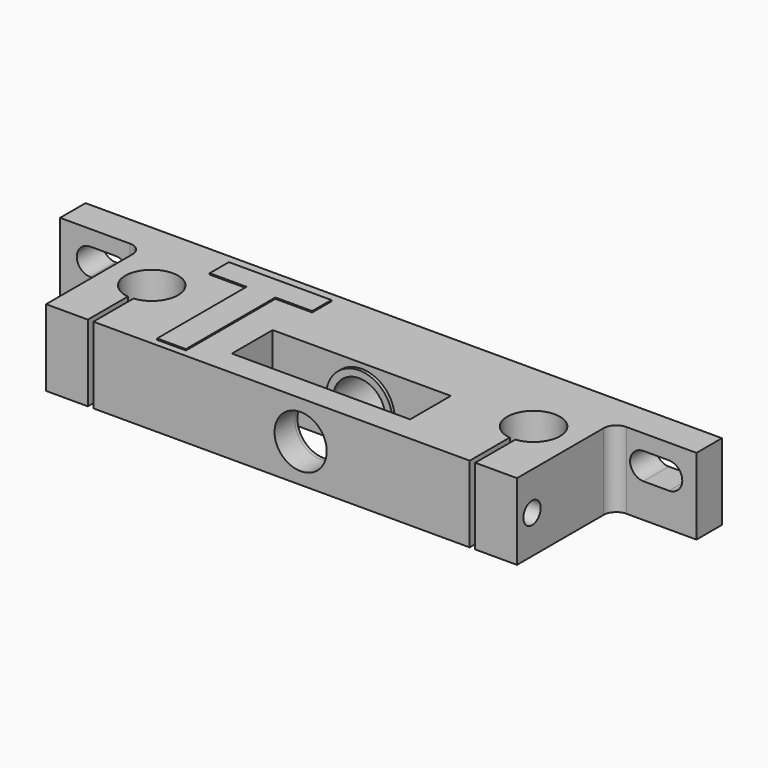
from build123d import *
from build123d import SkipClean  # not in build123d's __all__

# Parameters (mm, degrees)
F1_DEPTH      = 12
F3_DEPTH      = 12.001
F5_DEPTH      = 24.001
F6_R          = 4.1
F7_DEPTH      = 20
F8_W          = 14
F8_H          = 8
F9_DEPTH      = 12.001
F10_R         = 5.1951476321
F10_R_2       = 4.1
F11_DEPTH     = 0.5
F12_R         = 5.2529872518
F12_R_2       = 4.1
F13_DEPTH     = 0.5
F14_TEXT_SIZE = 29.872882718
F15_DEPTH     = 0.2
F16_R         = 1.4
F17_DEPTH     = 18
F16_R_2       = 1.7
F18_DEPTH     = 6.5630027184
F19_R         = 2
F20_R         = 1.4
F21_DEPTH     = 18
F20_R_2       = 1.7
F22_DEPTH     = 6.5630027184
F23_R         = 2


# Not quite as in the source:
# - after a boolean that leaves OpenCascade's solid faulty, fix() repairs it
# - Text() gives the source's letters only with a copy of the font that has no kerning and outlines rounded to 1/6400 em; it was checked with that copy


with BuildPart() as f1:
    # F0 (on Top) → F1 (new body)
    with BuildSketch(Plane.XY):
        Polygon((53.6500561982, 12.3083528318), (-46.3499438018, 12.3083528318), (-46.3499438018, 7.3083528318), (-33.3499438018, 7.3083528318), (-33.3499438018, -11.6916471682), (40.6500561982, -11.6916471682), (40.6500561982, 7.3083528318), (53.6500561982, 7.3083528318), align=None)
    extrude(amount=F1_DEPTH)

    # F2 (on face) → F3 (cut, through all)
    with BuildSketch(Plane.XY.offset(12)):
        with BuildLine():
            ThreePointArc((-25.9119465202, -3.818468994), (-23.2644787867, -2.4669679859), (-22.1999438018, 0.3083528318))
            ThreePointArc((-22.1999438018, 0.3083528318), (-29.1252646194, 3.3938178468), (-26.7879410833, -3.818468994))
            Line((-26.7879410833, -3.818468994), (-26.7879410833, -3.0108469723))
            Line((-26.7879410833, -3.0108469723), (-25.9119465202, -3.0108469723))
            Line((-25.9119465202, -3.0108469723), (-25.9119465202, -3.818468994))
        make_face()
        with BuildLine():
            Line((-26.7879410833, -3.0108469723), (-26.7879410833, -3.818468994))
            ThreePointArc((-26.7879410833, -3.818468994), (-26.3499438018, -3.8416471682), (-25.9119465202, -3.818468994))
            Line((-25.9119465202, -3.818468994), (-25.9119465202, -3.0108469723))
            Line((-25.9119465202, -3.0108469723), (-26.7879410833, -3.0108469723))
        make_face()
        with BuildLine():
            ThreePointArc((-25.9119465202, -3.818468994), (-26.3499438018, -3.8416471682), (-26.7879410833, -3.818468994))
            Line((-26.7879410833, -3.818468994), (-26.7879410833, -12.2696550748))
            Line((-26.7879410833, -12.2696550748), (-25.9119465202, -12.2696550748))
            Line((-25.9119465202, -12.2696550748), (-25.9119465202, -3.818468994))
        make_face()
        with BuildLine():
            ThreePointArc((34.0880534798, -3.818468994), (36.7355212133, -2.4669679859), (37.8000561982, 0.3083528318))
            ThreePointArc((37.8000561982, 0.3083528318), (30.8747353806, 3.3938178468), (33.2120589167, -3.818468994))
            Line((33.2120589167, -3.818468994), (33.2120589167, -3.0108469723))
            Line((33.2120589167, -3.0108469723), (34.0880534798, -3.0108469723))
            Line((34.0880534798, -3.0108469723), (34.0880534798, -3.818468994))
        make_face()
        with BuildLine():
            Line((33.2120589167, -3.0108469723), (33.2120589167, -3.818468994))
            ThreePointArc((33.2120589167, -3.818468994), (33.6500561982, -3.8416471682), (34.0880534798, -3.818468994))
            Line((34.0880534798, -3.818468994), (34.0880534798, -3.0108469723))
            Line((34.0880534798, -3.0108469723), (33.2120589167, -3.0108469723))
        make_face()
        with BuildLine():
            ThreePointArc((34.0880534798, -3.818468994), (33.6500561982, -3.8416471682), (33.2120589167, -3.818468994))
            Line((33.2120589167, -3.818468994), (33.2120589167, -12.2696550748))
            Line((33.2120589167, -12.2696550748), (34.0880534798, -12.2696550748))
            Line((34.0880534798, -12.2696550748), (34.0880534798, -3.818468994))
        make_face()
    extrude(amount=-F3_DEPTH, mode=Mode.SUBTRACT)

    # F4 (on face) → F5 (cut, through all)
    with BuildSketch(Plane(origin=(0, 12.3083528318, 0), x_dir=(-1, 0, 0), z_dir=(0, 1, 0))):
        with BuildLine():
            Line((-45.3214800954, 9.5596171677), (-49.3214800954, 9.5596171677))
            ThreePointArc((-49.3214800954, 9.5596171677), (-51.4214800954, 7.4596171677), (-49.3214800954, 5.3596171677))
            Line((-49.3214800954, 5.3596171677), (-45.3214800954, 5.3596171677))
            ThreePointArc((-45.3214800954, 5.3596171677), (-43.2214800954, 7.4596171677), (-45.3214800954, 9.5596171677))
        make_face()
        with BuildLine():
            ThreePointArc((37.6219116151, 9.5596171677), (35.5219116151, 7.4596171677), (37.6219116151, 5.3596171677))
            Line((37.6219116151, 5.3596171677), (41.6219116151, 5.3596171677))
            ThreePointArc((41.6219116151, 5.3596171677), (43.7219116151, 7.4596171677), (41.6219116151, 9.5596171677))
            Line((41.6219116151, 9.5596171677), (37.6219116151, 9.5596171677))
        make_face()
    extrude(amount=-F5_DEPTH, mode=Mode.SUBTRACT)

    # F6 (on face) → F7 (cut)
    with BuildSketch(Plane.XZ.offset(11.6916471682)):
        with Locations((6.6500561982, 6)):
            Circle(F6_R)
    extrude(amount=-F7_DEPTH, mode=Mode.SUBTRACT)

    # F8 (on face) → F9 (cut, through all)
    with BuildSketch(Plane.XY.offset(12)):
        with Locations((-0.3499438018, -3.6916471682)):
            Rectangle(F8_W, F8_H)
        with Locations((13.6500561982, -3.6916471682)):
            Rectangle(F8_W, F8_H)
    extrude(amount=-F9_DEPTH, mode=Mode.SUBTRACT)

    # F10 (on face) → F11 (join)
    with BuildSketch(Plane.XZ.offset(-0.3083528318)):
        with Locations((6.6500561982, 6)):
            Circle(F10_R)
        with Locations((6.6500561982, 6)):
            Circle(F10_R_2, mode=Mode.SUBTRACT)
    extrude(amount=F11_DEPTH)

    # F12 (on face) → F13 (join)
    with BuildSketch(Plane(origin=(0, -7.6916471682, 0), x_dir=(-1, 0, 0), z_dir=(0, 1, 0))):
        with Locations((-6.6500561982, 6)):
            Circle(F12_R)
        with Locations((-6.6500561982, 6)):
            Circle(F12_R_2, mode=Mode.SUBTRACT)
    with SkipClean():  # cleaning this boolean's faces spoils the solid; the shape is the same uncleaned
        extrude(amount=F13_DEPTH)

    # F14 (on face) → F15 (join)
    with BuildSketch(Plane.XY.offset(12)):
        with Locations((-23.175729205, -10.579360119)):
            Text('T', F14_TEXT_SIZE, font='Open Sans', font_style=FontStyle.BOLD, text_align=(TextAlign.LEFT, TextAlign.BOTTOM))
    extrude(amount=F15_DEPTH)

    add(f1.part.fix(), mode=Mode.REPLACE)

    # F16 (on face) → F17 (cut)
    with BuildSketch(Plane.YZ.offset(40.6500561982)):
        with Locations((-8.7363375351, 6)):
            Circle(F16_R)
    extrude(amount=-F17_DEPTH, mode=Mode.SUBTRACT)

    # F16 (on face) → F18 (cut, through all)
    with BuildSketch(Plane.YZ.offset(40.6500561982)):
        with Locations((-8.7363375351, 6)):
            Circle(F16_R_2)
        with Locations((-8.7363375351, 6)):
            Circle(F16_R, mode=Mode.SUBTRACT)
        with Locations((-8.7363375351, 6)):
            Circle(F16_R)
    extrude(amount=-F18_DEPTH, mode=Mode.SUBTRACT)

    # F19
    f19_edges = [f1.edges().sort_by_distance(p)[0] for p in [
        (40.650056, 7.308353, 6),
    ]]
    fillet(f19_edges, radius=F19_R)

    # F20 (on face) → F21 (cut)
    with BuildSketch(Plane(origin=(-33.3499438018, 0, 0), x_dir=(0, -1, 0), z_dir=(-1, 0, 0))):
        with Locations((8.7602175772, 6.004051771)):
            Circle(F20_R)
    extrude(amount=-F21_DEPTH, mode=Mode.SUBTRACT)

    # F20 (on face) → F22 (cut, through all)
    with BuildSketch(Plane(origin=(-33.3499438018, 0, 0), x_dir=(0, -1, 0), z_dir=(-1, 0, 0))):
        with Locations((8.7602175772, 6.004051771)):
            Circle(F20_R_2)
        with Locations((8.7602175772, 6.004051771)):
            Circle(F20_R, mode=Mode.SUBTRACT)
        with Locations((8.7602175772, 6.004051771)):
            Circle(F20_R)
    extrude(amount=-F22_DEPTH, mode=Mode.SUBTRACT)

    # F23
    f23_edges = [f1.edges().sort_by_distance(p)[0] for p in [
        (-33.349944, 7.308353, 6),
    ]]
    fillet(f23_edges, radius=F23_R)


solid = f1.part
